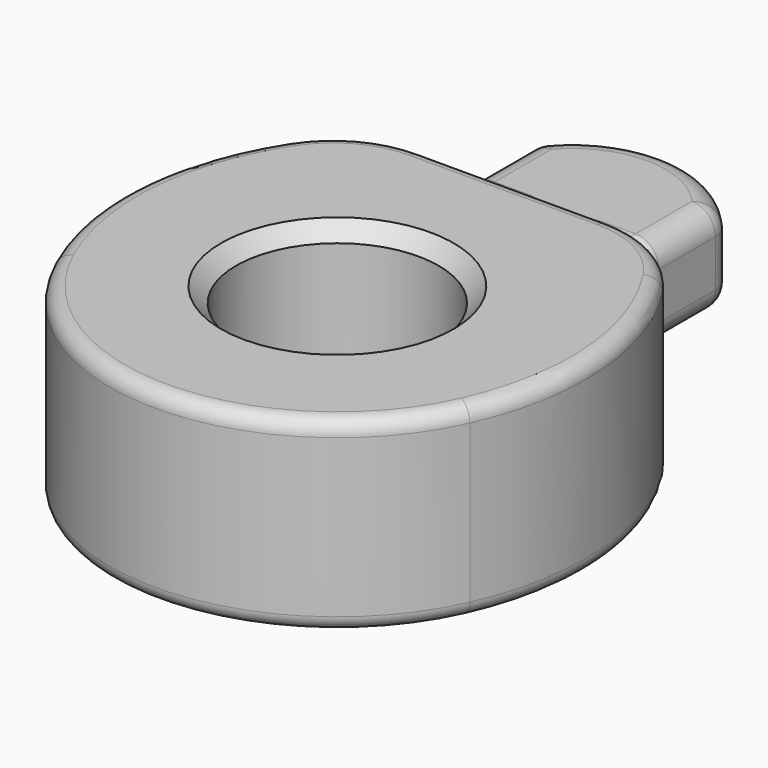
from build123d import *

# Parameters (mm, degrees)
F1_DEPTH = 1.5875
F2_DEPTH = 3.175
F3_R     = 3.17499
F4_R     = 0.79375
F6_DEPTH = 3.175
F7_R     = 0.508
F8_R     = 0.508
F9_SIZE  = 0.508


# Not quite as in the source:
# - a fillet or chamfer is up to 0.001 mm smaller than in the source, because OpenCascade refuses the exact size
# - a feature names something its author has since deleted; it is built from what else it names


with BuildPart() as f1:
    # F0 (on Top) → F1 (new body, symmetric)
    with BuildSketch(Plane.XY):
        with BuildLine():
            Line((3.175, 4.7625), (3.175, 7.9375))
            ThreePointArc((3.175, 7.9375), (0, 9.525), (-3.175, 7.9375))
            Line((-3.175, 7.9375), (-3.175, 4.7625))
            Line((-3.175, 4.7625), (-1.5875, 4.7625))
            Line((-1.5875, 4.7625), (-1.5875, 3.175))
            Line((-1.5875, 3.175), (1.5875, 3.175))
            Line((1.5875, 3.175), (1.5875, 4.7625))
            Line((1.5875, 4.7625), (3.175, 4.7625))
        make_face()
    extrude(amount=F1_DEPTH, both=True)

    # F0 (on Top) → F2 (join, symmetric)
    with BuildSketch(Plane.XY):
        Polygon((6.35, 3.175), (1.5875, 3.175), (-1.5875, 3.175), (-6.35, 3.175), (-6.35, 0), (6.35, 0), align=None)
    extrude(amount=F2_DEPTH, both=True)

    # F3 (radius 3.175 in the source; OpenCascade refuses exactly that, so slightly less here)
    f3_edges = [f1.edges().sort_by_distance(p)[0] for p in [
        (6.35, 3.175, 0),
        (-6.35, 3.175, 0),
    ]]
    fillet(f3_edges, radius=F3_R)

    # F4
    f4_edges = [f1.edges().sort_by_distance(p)[0] for p in [
        (0, 9.525, -1.5875),
        (0, 9.525, 1.5875),
        (3.175, 6.35, -1.5875),
        (3.175, 6.35, 1.5875),
        (-3.175, 6.35, -1.5875),
        (-3.175, 6.35, 1.5875),
        (3.175, 7.9375, 0),
        (-3.175, 7.9375, 0),
    ]]
    fillet(f4_edges, radius=F4_R)

    # F5 (on Top) → F6 (join, symmetric)
    with BuildSketch(Plane.XY):
        with BuildLine():
            Line((1.5875, 3.175), (-1.5875, 3.175))
            ThreePointArc((-1.5875, 3.175), (-6.8727430801, -0.8804299989), (-7.0214355114, -7.540625))
            ThreePointArc((-7.0214355114, -7.540625), (0, -12.0715436111), (7.0214355114, -7.540625))
            ThreePointArc((7.0214355114, -7.540625), (6.8727430801, -0.8804299989), (1.5875, 3.175))
        make_face()
        with BuildLine():
            ThreePointArc((0, -0.936625), (3.429, -4.365625), (0, -7.794625))
            ThreePointArc((0, -7.794625), (-3.429, -4.365625), (0, -0.936625))
        make_face(mode=Mode.SUBTRACT)
        with BuildLine():
            Line((3.175, 3.175), (1.5875, 3.175))
            ThreePointArc((1.5875, 3.175), (6.8727430801, -0.8804299989), (7.0214355114, -7.540625))
            ThreePointArc((7.0214355114, -7.540625), (7.829384353, -2.9521060097), (6.3352448193, 1.4609241182))
            ThreePointArc((6.3352448193, 1.4609241182), (4.9725819485, 2.7188926062), (3.175, 3.175))
        make_face()
        with BuildLine():
            Line((-1.5875, 3.175), (-3.175, 3.175))
            ThreePointArc((-3.175, 3.175), (-4.9725819485, 2.7188926062), (-6.3352448193, 1.4609241182))
            ThreePointArc((-6.3352448193, 1.4609241182), (-7.829384353, -2.9521060097), (-7.0214355114, -7.540625))
            ThreePointArc((-7.0214355114, -7.540625), (-6.8727430801, -0.8804299989), (-1.5875, 3.175))
        make_face()
    extrude(amount=F6_DEPTH, both=True)

    # F7
    f7_edges = [f1.edges().sort_by_distance(p)[0] for p in [
        (0, 3.175, -1.5875),
        (-1.5875, 3.175, 0),
        (0, 3.175, 1.5875),
        (1.5875, 3.175, 0),
        (1.5875, 3.96875, 1.5875),
        (1.5875, 3.96875, -1.5875),
        (-1.5875, 3.96875, -1.5875),
        (-1.5875, 3.96875, 1.5875),
        (2.942516, 4.7625, 1.355016),
        (-2.942516, 4.7625, -1.355016),
    ]]
    fillet(f7_edges, radius=F7_R)

    # F8
    f8_edges = [f1.edges().sort_by_distance(p)[0] for p in [
        (-7.829384, -2.952106, -3.175),
        (-7.829384, -2.952106, 3.175),
        (0, 3.175, -3.175),
        (0, 3.175, 3.175),
        (-4.972586, 2.71889, -3.175),
        (0, -12.071544, -3.175),
        (7.829384, -2.952106, -3.175),
        (4.972586, 2.71889, -3.175),
        (4.972586, 2.71889, 3.175),
        (-4.972586, 2.71889, 3.175),
        (0, -12.071544, 3.175),
        (7.829384, -2.952106, 3.175),
    ]]
    fillet(f8_edges, radius=F8_R)

    # F9
    f9_edges = [f1.edges().sort_by_distance(p)[0] for p in [
        (0, -0.936625, 3.175),
        (0, -0.936625, -3.175),
    ]]
    chamfer(f9_edges, length=F9_SIZE)


solid = f1.part
